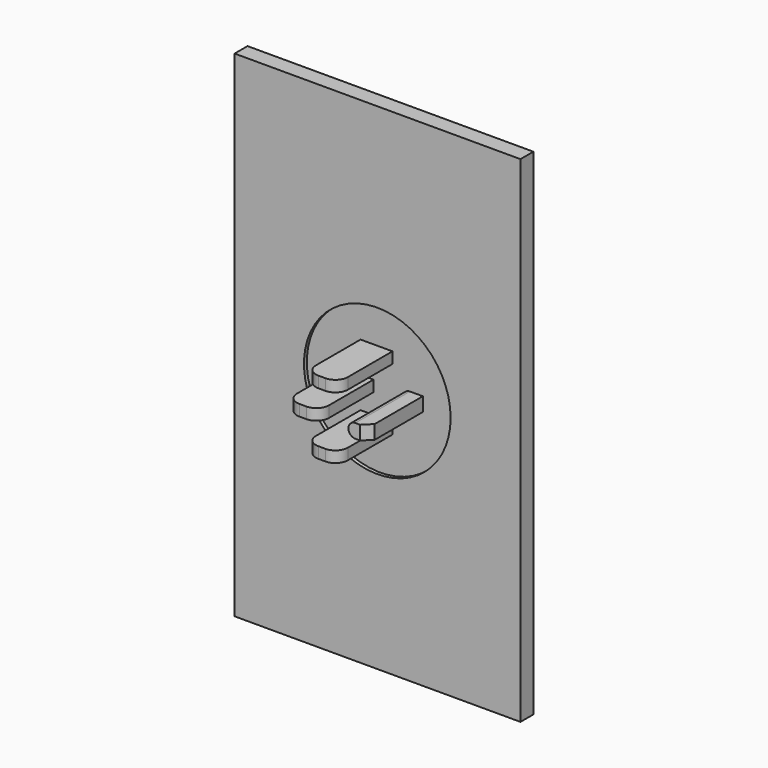
from build123d import *

# Parameters (mm, degrees)
F0_W     = 88.39527
F0_H     = 153.20968
F0_R     = 22.6744372739
F1_DEPTH = 5
F0_W_2   = 9.8689098377
F0_H_2   = 3.4395875409
F0_W_3   = 9.86891
F0_H_3   = 3.43959
F2_DEPTH = 3.9
F3_DEPTH = 25
F4_R     = 3.8627416998
F5_SIZE  = 2.5


# Not quite as in the source:
# - a feature names something its author has since deleted; it is built from what else it names


with BuildPart() as f1:
    # F0 (on Front) → F1 (new body)
    with BuildSketch(Plane.XZ):
        with Locations((4.9840081745, 0.7166508444)):
            Rectangle(F0_W, F0_H)
        with Locations((4.9144495279, -0.1638149843)):
            Circle(F0_R, mode=Mode.SUBTRACT)
    extrude(amount=F1_DEPTH)

    # F0 (on Front) → F2 (join)
    with BuildSketch(Plane.XZ):
        with Locations((4.9144495279, -0.1638149843)):
            Circle(F0_R)
        with Locations((3.791642841, -9.5432697745)):
            Rectangle(F0_W_2, F0_H_2, mode=Mode.SUBTRACT)
        with Locations((-2.0837161803, 0.0662026977)):
            Rectangle(F0_W_3, F0_H_3, mode=Mode.SUBTRACT)
        with BuildLine():
            Line((18.1140358327, 2.2190151321), (18.1140358327, -2.0737481719))
            Line((18.1140358327, -2.0737481719), (14.117325074, -2.0737481719))
            ThreePointArc((14.117325074, -2.0737481719), (11.9709434221, 0.0726334801), (14.117325074, 2.2190151321))
            Line((14.117325074, 2.2190151321), (18.1140358327, 2.2190151321))
        make_face(mode=Mode.SUBTRACT)
        with Locations((3.791642841, 9.6756751699)):
            Rectangle(F0_W_2, F0_H_2, mode=Mode.SUBTRACT)
    extrude(amount=F2_DEPTH)

    # F0 (on Front) → F3 (join)
    with BuildSketch(Plane.XZ):
        with Locations((3.791642841, -9.5432697745)):
            Rectangle(F0_W_2, F0_H_2)
        with Locations((-2.0837161803, 0.0662026977)):
            Rectangle(F0_W_3, F0_H_3)
        with Locations((3.791642841, 9.6756751699)):
            Rectangle(F0_W_2, F0_H_2)
        with BuildLine():
            Line((14.117325074, -2.0737481719), (18.1140358327, -2.0737481719))
            Line((18.1140358327, -2.0737481719), (18.1140358327, 2.2190151321))
            Line((18.1140358327, 2.2190151321), (14.117325074, 2.2190151321))
            ThreePointArc((14.117325074, 2.2190151321), (11.9709434221, 0.0726334801), (14.117325074, -2.0737481719))
        make_face()
    extrude(amount=F3_DEPTH)

    # F4
    f4_edges = [f1.edges().sort_by_distance(p)[0] for p in [
        (-1.142812, -25, -9.54327),
        (8.726098, -25, -9.54327),
        (-7.018171, -25, 0.066203),
        (2.850739, -25, 0.066203),
        (8.726098, -25, 9.675675),
        (-1.142812, -25, 9.675675),
    ]]
    fillet(f4_edges, radius=F4_R)

    # F5
    f5_edges = [f1.edges().sort_by_distance(p)[0] for p in [
        (18.114036, -25, 0.072633),
    ]]
    chamfer(f5_edges, length=F5_SIZE)


solid = f1.part
